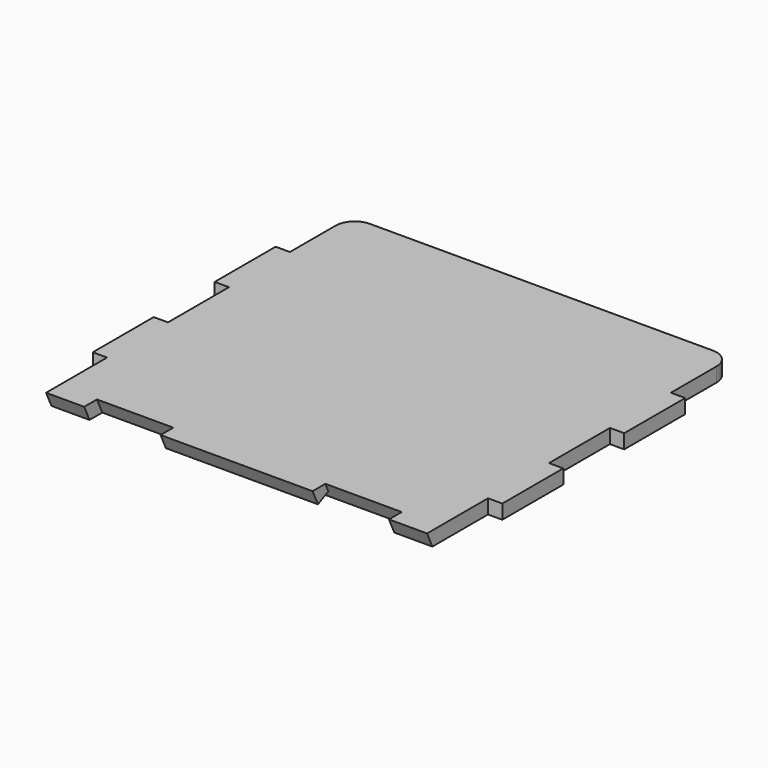
from build123d import *

# Parameters (mm, degrees)
F1_DEPTH  = 19.05
F2_R      = 25.4
F4_DEPTH  = 527.051
F6_W      = 101.854
F6_H      = 19.2786
F7_DEPTH  = 231.9562403073
F9_W      = 202.692
F9_H      = 19.2786
F10_DEPTH = 210.9250403073


with BuildPart() as f1:
    # F0 (on Top) → F1 (new body)
    with BuildSketch(Plane.XY):
        Polygon((0, 101.6), (0, 0), (508, 0), (508, 101.6), (527.05, 101.6), (527.05, 152.4), (527.05, 203.2), (508, 203.2), (508, 304.8), (527.05, 304.8), (527.05, 355.6), (527.05, 406.4), (508, 406.4), (508, 508), (254, 508), (0, 508), (0, 406.4), (-19.05, 406.4), (-19.05, 355.6), (-19.05, 304.8), (0, 304.8), (0, 203.2), (-19.05, 203.2), (-19.05, 152.4), (-19.05, 101.6), align=None)
    extrude(amount=F1_DEPTH)

    # F2
    f2_edges = [f1.edges().sort_by_distance(p)[0] for p in [
        (0, 508, 9.525),
        (508, 508, 9.525),
    ]]
    fillet(f2_edges, radius=F2_R)

    # F3 (on face) → F4 (cut, through all)
    with BuildSketch(Plane(origin=(0, 0, 0), x_dir=(0, -1, 0), z_dir=(-1, 0, 0))):
        Polygon((0, 0), (0, 19.05), (-8.8831608879, 0), align=None)
    extrude(amount=-F4_DEPTH, mode=Mode.SUBTRACT)

    # F6 (on face) → F7 (cut, through all)
    with BuildSketch(Plane(origin=(0, -7.2965733207, 15.6475519823), x_dir=(1, 0, 0), z_dir=(0, 0.4226182617, -0.906307787))):
        with Locations((101.727, -17.6901778862)):
            Rectangle(F6_W, F6_H)
        with Locations((406.273, -17.6901778862)):
            Rectangle(F6_W, F6_H)
    extrude(amount=F7_DEPTH, mode=Mode.SUBTRACT)

    # F9 (on face) → F10 (cut, through all)
    with BuildSketch(Plane(origin=(0, 1.5915958656, -3.4131883485), x_dir=(1, 0, 0), z_dir=(0, 0.4226182617, -0.906307787))):
        with Locations((254, -17.6901778862)):
            Rectangle(F9_W, F9_H)
    extrude(amount=F10_DEPTH, mode=Mode.SUBTRACT)


solid = f1.part
